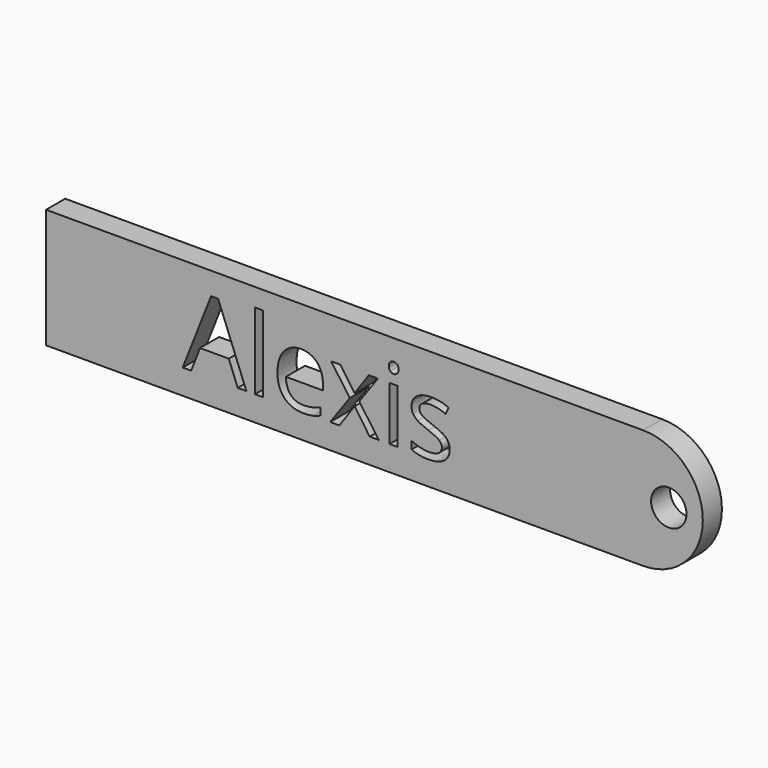
from build123d import *

# Parameters (mm, degrees)
F0_W     = 0.6829528259
F0_H     = 4.5069622906
F0_H_2   = 6.3992285019
F0_R     = 1.4814772489
F1_DEPTH = 2


with BuildPart() as f1:
    # F0 (on Front) → F1 (new body)
    with BuildSketch(Plane.XZ):
        with BuildLine():
            Line((15.6519781798, 28.567796193), (-34.3480218202, 28.567796193))
            Line((-34.3480218202, 28.567796193), (-34.3480218202, 18.567796193))
            Line((-34.3480218202, 18.567796193), (15.6519781798, 18.567796193))
            ThreePointArc((15.6519781798, 18.567796193), (20.6519781798, 23.567796193), (15.6519781798, 28.567796193))
        make_face()
        with BuildLine():
            add(Edge.make_bspline(
                [(-12.0378659954, 20.6372455488), (-12.3602618381, 20.5688186761), (-12.8168796234, 20.5688186761)],
                knots=[0, 0, 0, 1, 1, 1], degree=2))
            add(Edge.make_bspline(
                [(-12.8168796234, 20.5688186761), (-13.8156487851, 20.5688186761), (-14.3939874498, 21.1780810237)],
                knots=[0, 0, 0, 1, 1, 1], degree=2))
            add(Edge.make_bspline(
                [(-14.3939874498, 21.1780810237), (-14.9723261145, 21.7873433713), (-14.9723261145, 22.8676984197)],
                knots=[0, 0, 0, 1, 1, 1], degree=2))
            add(Edge.make_bspline(
                [(-14.9723261145, 22.8676984197), (-14.9723261145, 23.9585806792), (-14.4354383439, 24.6000826111)],
                knots=[0, 0, 0, 1, 1, 1], degree=2))
            add(Edge.make_bspline(
                [(-14.4354383439, 24.6000826111), (-13.8985505732, 25.2415845429), (-12.9932104109, 25.2415845429)],
                knots=[0, 0, 0, 1, 1, 1], degree=2))
            add(Edge.make_bspline(
                [(-12.9932104109, 25.2415845429), (-12.1470858115, 25.2415845429), (-11.653622787, 24.6843003006)],
                knots=[0, 0, 0, 1, 1, 1], degree=2))
            add(Edge.make_bspline(
                [(-11.653622787, 24.6843003006), (-11.1601597625, 24.1270160582), (-11.1601597625, 23.2137804875)],
                knots=[0, 0, 0, 1, 1, 1], degree=2))
            Line((-11.1601597625, 23.2137804875), (-11.1601597625, 22.7821648287))
            Line((-11.1601597625, 22.7821648287), (-14.264371162, 22.7821648287))
            add(Edge.make_bspline(
                [(-14.264371162, 22.7821648287), (-14.2433167396, 21.9886762853), (-13.8630212354, 21.5774570982)],
                knots=[0, 0, 0, 1, 1, 1], degree=2))
            add(Edge.make_bspline(
                [(-13.8630212354, 21.5774570982), (-13.4827257312, 21.1662379111), (-12.7918774969, 21.1662379111)],
                knots=[0, 0, 0, 1, 1, 1], degree=2))
            add(Edge.make_bspline(
                [(-12.7918774969, 21.1662379111), (-12.0641840234, 21.1662379111), (-11.3535972681, 21.4702111342)],
                knots=[0, 0, 0, 1, 1, 1], degree=2))
            Line((-11.3535972681, 21.4702111342), (-11.3535972681, 20.8609487866))
            add(Edge.make_bspline(
                [(-11.3535972681, 20.8609487866), (-11.7154701527, 20.7056724216), (-12.0378659954, 20.6372455488)],
                knots=[0, 0, 0, 1, 1, 1], degree=2))
        make_face(mode=Mode.SUBTRACT)
        Polygon((-10.5587928233, 20.6517204642), (-8.9099683707, 22.9584956162), (-10.4772069365, 25.1586827548), (-9.6995092099, 25.1586827548), (-8.5112502469, 23.4322201197), (-7.326938988, 25.1586827548), (-6.5571366698, 25.1586827548), (-8.1243752356, 22.9584956162), (-6.4755507831, 20.6517204642), (-7.2479849041, 20.6517204642), (-8.5112502469, 22.4781916056), (-9.7863587022, 20.6517204642), align=None, mode=Mode.SUBTRACT)
        with Locations((-5.2418932218, 22.9052016095)):
            Rectangle(F0_W, F0_H, mode=Mode.SUBTRACT)
        with BuildLine():
            add(Edge.make_bspline(
                [(-0.8277019798, 22.6255725623), (-0.5460990805, 22.3294947476), (-0.5460990805, 21.8807723706)],
                knots=[0, 0, 0, 1, 1, 1], degree=2))
            add(Edge.make_bspline(
                [(-0.5460990805, 21.8807723706), (-0.5460990805, 21.251771502), (-1.0145599784, 20.9102950891)],
                knots=[0, 0, 0, 1, 1, 1], degree=2))
            add(Edge.make_bspline(
                [(-1.0145599784, 20.9102950891), (-1.4830208763, 20.5688186761), (-2.3304613771, 20.5688186761)],
                knots=[0, 0, 0, 1, 1, 1], degree=2))
            add(Edge.make_bspline(
                [(-2.3304613771, 20.5688186761), (-3.2265902296, 20.5688186761), (-3.7279486625, 20.8530533782)],
                knots=[0, 0, 0, 1, 1, 1], degree=2))
            Line((-3.7279486625, 20.8530533782), (-3.7279486625, 21.486001951))
            add(Edge.make_bspline(
                [(-3.7279486625, 21.486001951), (-3.4029210171, 21.3215142762), (-3.0311788719, 21.2274273262)],
                knots=[0, 0, 0, 1, 1, 1], degree=2))
            add(Edge.make_bspline(
                [(-3.0311788719, 21.2274273262), (-2.6594367268, 21.1333403762), (-2.3133546589, 21.1333403762)],
                knots=[0, 0, 0, 1, 1, 1], degree=2))
            add(Edge.make_bspline(
                [(-2.3133546589, 21.1333403762), (-1.7790986911, 21.1333403762), (-1.4915742354, 21.3037496073)],
                knots=[0, 0, 0, 1, 1, 1], degree=2))
            add(Edge.make_bspline(
                [(-1.4915742354, 21.3037496073), (-1.2040497798, 21.4741588384), (-1.2040497798, 21.8241886105)],
                knots=[0, 0, 0, 1, 1, 1], degree=2))
            add(Edge.make_bspline(
                [(-1.2040497798, 21.8241886105), (-1.2040497798, 22.0873688902), (-1.4317007218, 22.2742268888)],
                knots=[0, 0, 0, 1, 1, 1], degree=2))
            add(Edge.make_bspline(
                [(-1.4317007218, 22.2742268888), (-1.6593516638, 22.4610848875), (-2.3225659687, 22.7163697588)],
                knots=[0, 0, 0, 1, 1, 1], degree=2))
            add(Edge.make_bspline(
                [(-2.3225659687, 22.7163697588), (-2.9515668373, 22.9506002078), (-3.2167209691, 23.1256150938)],
                knots=[0, 0, 0, 1, 1, 1], degree=2))
            add(Edge.make_bspline(
                [(-3.2167209691, 23.1256150938), (-3.481875101, 23.3006299798), (-3.6114913888, 23.5223593655)],
                knots=[0, 0, 0, 1, 1, 1], degree=2))
            add(Edge.make_bspline(
                [(-3.6114913888, 23.5223593655), (-3.7411076765, 23.7440887512), (-3.7411076765, 24.0520096785)],
                knots=[0, 0, 0, 1, 1, 1], degree=2))
            add(Edge.make_bspline(
                [(-3.7411076765, 24.0520096785), (-3.7411076765, 24.6033723646), (-3.2923852996, 24.9224784537)],
                knots=[0, 0, 0, 1, 1, 1], degree=2))
            add(Edge.make_bspline(
                [(-3.2923852996, 24.9224784537), (-2.8436629226, 25.2415845429), (-2.0633333932, 25.2415845429)],
                knots=[0, 0, 0, 1, 1, 1], degree=2))
            add(Edge.make_bspline(
                [(-2.0633333932, 25.2415845429), (-1.3356399197, 25.2415845429), (-0.6395280798, 24.9455067282)],
                knots=[0, 0, 0, 1, 1, 1], degree=2))
            Line((-0.6395280798, 24.9455067282), (-0.8829698385, 24.390196338))
            add(Edge.make_bspline(
                [(-0.8829698385, 24.390196338), (-1.5606590589, 24.6691674345), (-2.1120217449, 24.6691674345)],
                knots=[0, 0, 0, 1, 1, 1], degree=2))
            add(Edge.make_bspline(
                [(-2.1120217449, 24.6691674345), (-2.5975893611, 24.6691674345), (-2.8443208733, 24.5171808229)],
                knots=[0, 0, 0, 1, 1, 1], degree=2))
            add(Edge.make_bspline(
                [(-2.8443208733, 24.5171808229), (-3.0910523856, 24.3651942114), (-3.0910523856, 24.0980662275)],
                knots=[0, 0, 0, 1, 1, 1], degree=2))
            add(Edge.make_bspline(
                [(-3.0910523856, 24.0980662275), (-3.0910523856, 23.9164718344), (-2.998281337, 23.7894873495)],
                knots=[0, 0, 0, 1, 1, 1], degree=2))
            add(Edge.make_bspline(
                [(-2.998281337, 23.7894873495), (-2.9055102884, 23.6625028645), (-2.7002296702, 23.5473614921)],
                knots=[0, 0, 0, 1, 1, 1], degree=2))
            add(Edge.make_bspline(
                [(-2.7002296702, 23.5473614921), (-2.494949052, 23.4322201197), (-1.9106888309, 23.2137804875)],
                knots=[0, 0, 0, 1, 1, 1], degree=2))
            add(Edge.make_bspline(
                [(-1.9106888309, 23.2137804875), (-1.1093048791, 22.921650377), (-0.8277019798, 22.6255725623)],
                knots=[0, 0, 0, 1, 1, 1], degree=2))
        make_face(mode=Mode.SUBTRACT)
        Polygon((-17.5751790812, 20.6517204642), (-18.2989248505, 20.6517204642), (-19.0476727463, 22.5637251966), (-21.4570882074, 22.5637251966), (-22.1966247934, 20.6517204642), (-22.904579746, 20.6517204642), (-20.5280618199, 26.6890760815), (-19.9398538947, 26.6890760815), align=None, mode=Mode.SUBTRACT)
        with Locations((-16.5099568989, 23.8513347152)):
            Rectangle(F0_W, F0_H_2, mode=Mode.SUBTRACT)
        with Locations((17.7988428622, 23.567796193)):
            Circle(F0_R, mode=Mode.SUBTRACT)
        with BuildLine():
            add(Edge.make_bspline(
                [(-5.5261279239, 26.0363889878), (-5.6412692963, 26.149556508), (-5.6412692963, 26.3798392528)],
                knots=[0, 0, 0, 1, 1, 1], degree=2))
            add(Edge.make_bspline(
                [(-5.6412692963, 26.3798392528), (-5.6412692963, 26.6140697018), (-5.5261279239, 26.7232895179)],
                knots=[0, 0, 0, 1, 1, 1], degree=2))
            add(Edge.make_bspline(
                [(-5.5261279239, 26.7232895179), (-5.4109865515, 26.832509334), (-5.2372875669, 26.832509334)],
                knots=[0, 0, 0, 1, 1, 1], degree=2))
            add(Edge.make_bspline(
                [(-5.2372875669, 26.832509334), (-5.072799892, 26.832509334), (-4.9537108154, 26.7213156658)],
                knots=[0, 0, 0, 1, 1, 1], degree=2))
            add(Edge.make_bspline(
                [(-4.9537108154, 26.7213156658), (-4.8346217389, 26.6101219976), (-4.8346217389, 26.3798392528)],
                knots=[0, 0, 0, 1, 1, 1], degree=2))
            add(Edge.make_bspline(
                [(-4.8346217389, 26.3798392528), (-4.8346217389, 26.149556508), (-4.9537108154, 26.0363889878)],
                knots=[0, 0, 0, 1, 1, 1], degree=2))
            add(Edge.make_bspline(
                [(-4.9537108154, 26.0363889878), (-5.072799892, 25.9232214675), (-5.2372875669, 25.9232214675)],
                knots=[0, 0, 0, 1, 1, 1], degree=2))
            add(Edge.make_bspline(
                [(-5.2372875669, 25.9232214675), (-5.4109865515, 25.9232214675), (-5.5261279239, 26.0363889878)],
                knots=[0, 0, 0, 1, 1, 1], degree=2))
        make_face(mode=Mode.SUBTRACT)
    extrude(amount=F1_DEPTH)


solid = f1.part
